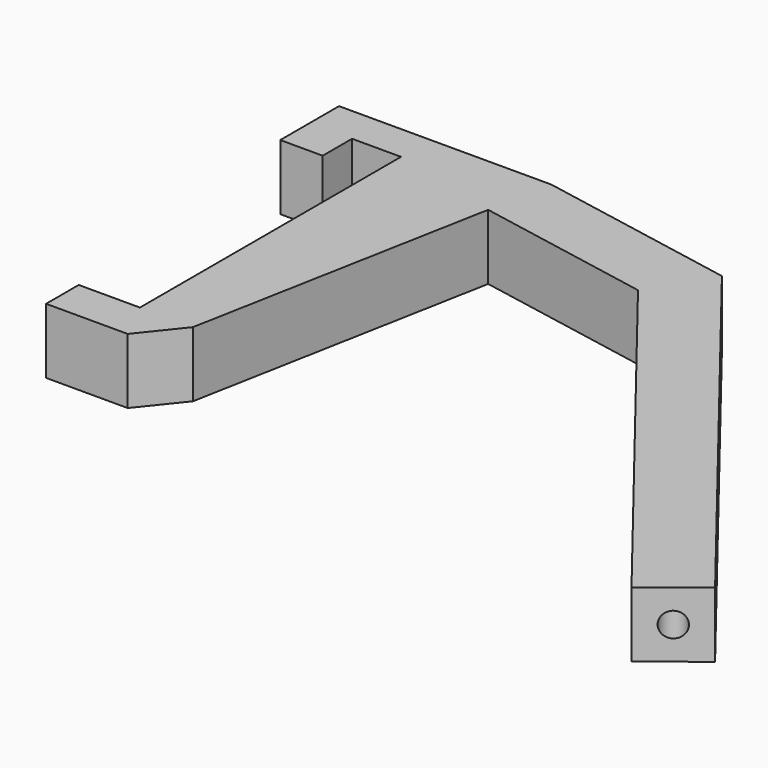
from build123d import *

# Parameters (mm, degrees)
F1_DEPTH = 8
F3_D     = 3
F3_DEPTH = 6
F3_TIP   = 0.9012909285


with BuildPart() as f1:
    # F0 (on Top) → F1 (new body)
    with BuildSketch(Plane.XY):
        Polygon((-35.0272064194, 47.1324694753), (-35.0272064194, 51.6324694753), (-29.0272064194, 51.6324694753), (-29.0272064194, 11.6324694753), (-36.5272064194, 11.6324694753), (-36.5272064194, 6.6324694753), (-26.5272064194, 6.6324694753), (-22.5272064194, 11.6324694753), (-15.6577646998, 48.2694919798), (5.9506252409, 44.2179188659), (43.934325687, -4.2605536739), (50.2315890367, 0.6734583148), (10.388348254, 51.525256099), (-14.1834564194, 56.1324694753), (-40.2272064194, 56.1324694753), (-40.2272064194, 47.1324694753), align=None)
    extrude(amount=F1_DEPTH)

    # F3
    with Locations(Plane(origin=(18.7802618476, -23.969186719, 0), x_dir=(0.7871579187, 0.6167514986, 0), z_dir=(0.6167514986, -0.7871579187, 0))):
        with Locations((35.9555495046, 4)):
            Hole(F3_D / 2, depth=F3_DEPTH)
            with Locations((0, 0, -(F3_DEPTH + F3_TIP / 2))):  # 118° drill point
                Cone(0, F3_D / 2, F3_TIP, mode=Mode.SUBTRACT)


solid = f1.part
